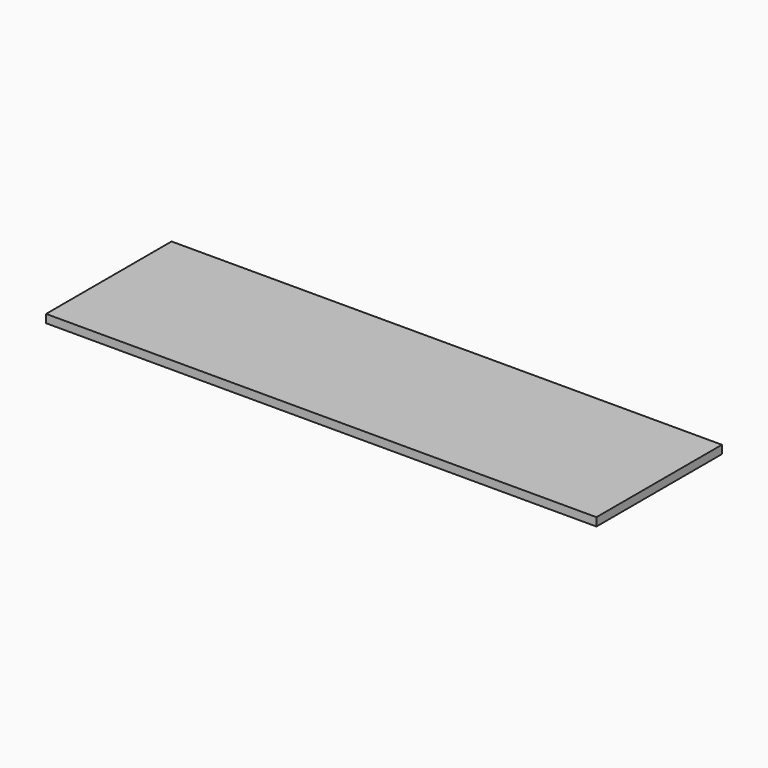
from build123d import *

# Parameters (mm, degrees)
F1_DEPTH = 3


# Not quite as in the source:
# - the program builds the solid bodies; features that only make, move or delete a surface that nothing else refers to are left out


with BuildPart() as f1:
    # F0 (on Top) → F1 (new body)
    with BuildSketch(Plane.XY):
        Polygon((74.5923221111, 0), (0, 0), (0, -56.9987312751), (200, -56.9987312751), (200, 0), (114.5923221111, 0), align=None)
    extrude(amount=F1_DEPTH)


solid = f1.part
